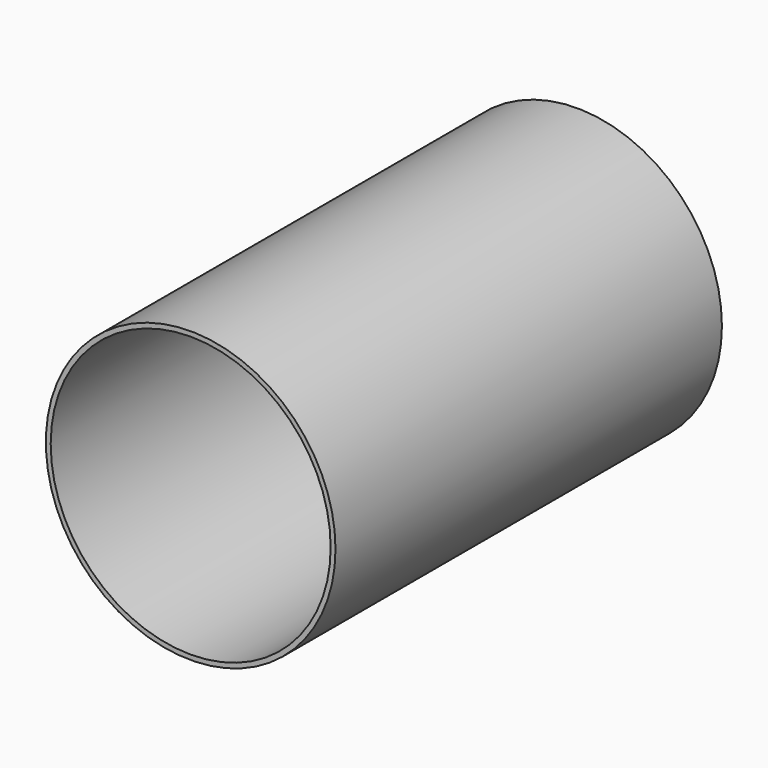
from build123d import *

# Parameters (mm, degrees)
F0_R         = 76.1481947207
F1_DEPTH     = 254
F2_T         = -2.54
F3_TEXT_SIZE = 21.7371115771
F4_DEPTH     = 25.4


# Not quite as in the source:
# - Text() gives the source's letters only with a copy of the font that has no kerning and outlines rounded to 1/6400 em; it was checked with that copy


with BuildPart() as f1:
    # F0 (on Front) → F1 (new body)
    with BuildSketch(Plane.XZ):
        Circle(F0_R)
    extrude(amount=F1_DEPTH)

    # F2
    f2_openings = [f1.faces().sort_by_distance(p)[0] for p in [
        (0, -254, 0),
    ]]
    offset(amount=F2_T, openings=f2_openings)

    # F3 (on face) → F4 (cut)
    with BuildSketch(Plane.XZ.offset(2.54)):
        with Locations((-38.2547527552, -7.5121093541)):
            Text('M.G', F3_TEXT_SIZE, font='Open Sans', text_align=(TextAlign.LEFT, TextAlign.BOTTOM))
    extrude(amount=-F4_DEPTH, mode=Mode.SUBTRACT)


solid = f1.part
